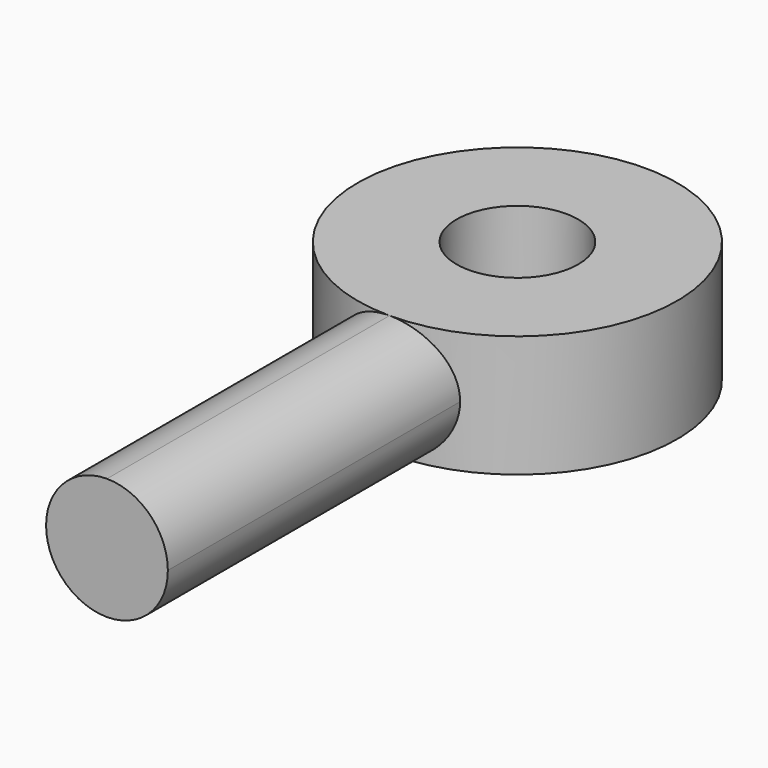
from build123d import *

# Parameters (mm, degrees)
F0_R     = 6.35
F1_DEPTH = 6.35
F2_R     = 6.34999


# Not quite as in the source:
# - a fillet or chamfer is up to 0.001 mm smaller than in the source, because OpenCascade refuses the exact size


with BuildPart() as f1:
    # F0 (on Top) → F1 (new body, symmetric)
    with BuildSketch(Plane.XY):
        with BuildLine():
            ThreePointArc((6.35, -15.4118372222), (0, 16.66875), (-6.35, -15.4118372222))
            Line((-6.35, -15.4118372222), (-6.35, -53.5118372222))
            Line((-6.35, -53.5118372222), (6.35, -53.5118372222))
            Line((6.35, -53.5118372222), (6.35, -15.4118372222))
        make_face()
        Circle(F0_R, mode=Mode.SUBTRACT)
    extrude(amount=F1_DEPTH, both=True)

    # F2 (radius 6.35 in the source; OpenCascade refuses exactly that, so slightly less here)
    f2_edges = [f1.edges().sort_by_distance(p)[0] for p in [
        (-6.35, -34.461837, -6.35),
        (6.35, -34.461837, -6.35),
        (-6.35, -34.461837, 6.35),
        (6.35, -34.461837, 6.35),
    ]]
    fillet(f2_edges, radius=F2_R)


solid = f1.part
